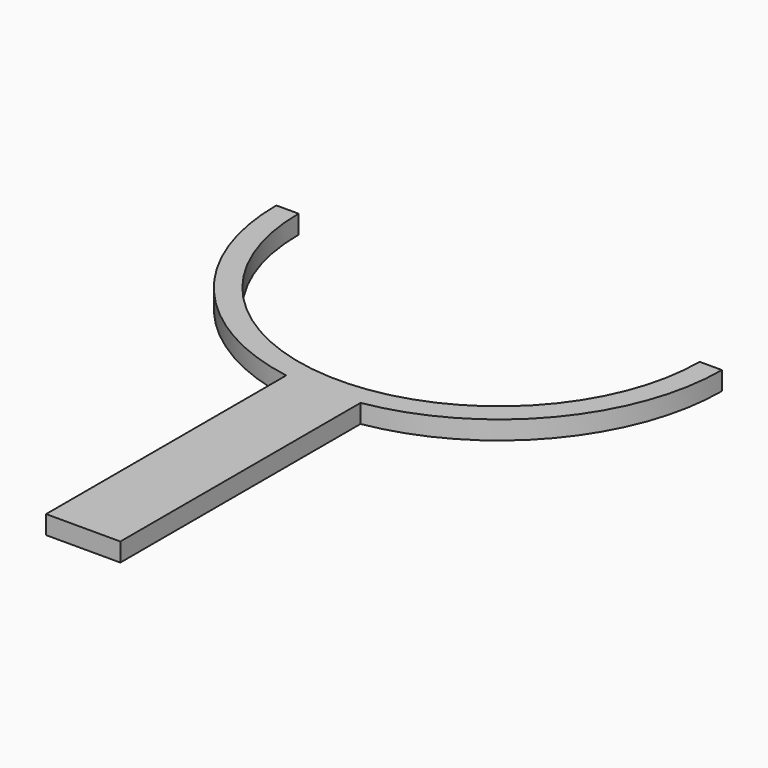
from build123d import *

# Parameters (mm, degrees)
F1_DEPTH = 3.175


# Not quite as in the source:
# - a feature names something its author has since deleted; it is built from what else it names


with BuildPart() as f1:
    # F0 (on Top) → F1 (new body)
    with BuildSketch(Plane.XY):
        with BuildLine():
            Line((-6.35, 25.4), (-6.35, -25.4))
            Line((-6.35, -25.4), (6.35, -25.4))
            Line((6.35, -25.4), (6.35, 25.4))
            Line((6.35, 25.4), (6.35, 25.9328933773))
            ThreePointArc((6.35, 25.9328933773), (0, 25.4), (-6.35, 25.9328933773))
            Line((-6.35, 25.9328933773), (-6.35, 25.4))
        make_face()
        with BuildLine():
            ThreePointArc((-38.1, 63.5), (-29.099355663, 38.9065557516), (-6.35, 25.9328933773))
            ThreePointArc((-6.35, 25.9328933773), (0, 25.4), (6.35, 25.9328933773))
            ThreePointArc((6.35, 25.9328933773), (29.099355663, 38.9065557516), (38.1, 63.5))
            Line((38.1, 63.5), (34.29, 63.5))
            ThreePointArc((34.29, 63.5), (0, 29.21), (-34.29, 63.5))
            Line((-34.29, 63.5), (-38.1, 63.5))
        make_face()
    extrude(amount=F1_DEPTH)


solid = f1.part
